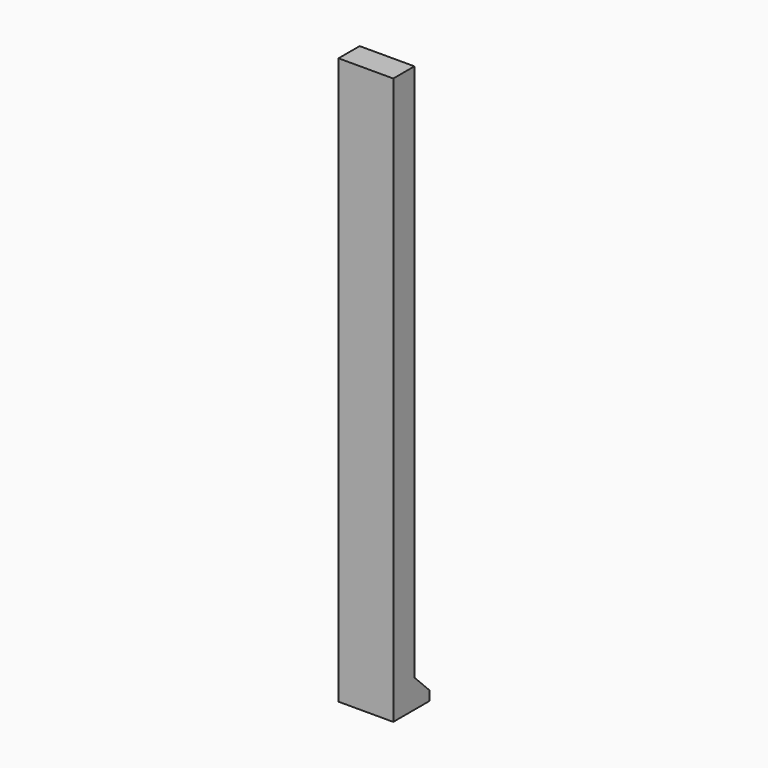
from build123d import *

# Parameters (mm, degrees)
F0_W     = 5.8
F0_H     = 2
F0_H_2   = 2.8
F1_DEPTH = 3
F2_DEPTH = 60
F3_SIZE  = 1.99999


# Not quite as in the source:
# - a fillet or chamfer is up to 0.001 mm smaller than in the source, because OpenCascade refuses the exact size
# - a feature names something its author has since deleted; it is built from what else it names


with BuildPart() as f1:
    # F0 (on Top) → F1 (new body)
    with BuildSketch(Plane.XY):
        with Locations((-14.8613960065, 7.2783571027)):
            Rectangle(F0_W, F0_H)
        with Locations((-14.8613960065, 4.8783571027)):
            Rectangle(F0_W, F0_H_2)
    extrude(amount=F1_DEPTH)

    # F0 (on Top) → F2 (join)
    with BuildSketch(Plane.XY):
        with Locations((-14.8613960065, 4.8783571027)):
            Rectangle(F0_W, F0_H_2)
    extrude(amount=F2_DEPTH)

    # F3 (size 2 in the source; OpenCascade refuses exactly that, so slightly less here)
    f3_edges = [f1.edges().sort_by_distance(p)[0] for p in [
        (-14.861396, 8.278357, 3),
    ]]
    chamfer(f3_edges, length=F3_SIZE)


solid = f1.part
